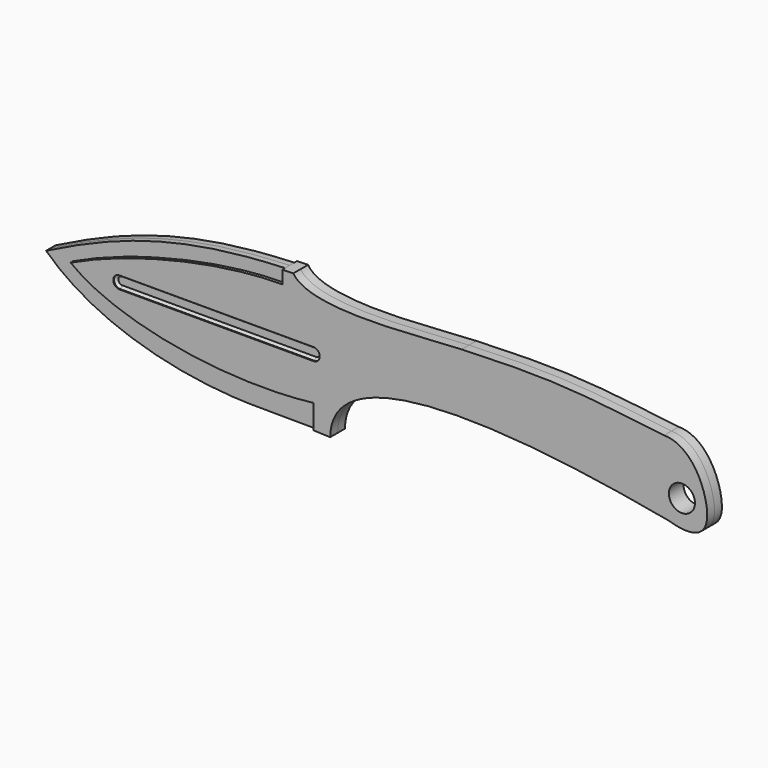
from build123d import *

# Parameters (mm, degrees)
F0_R     = 4.5078911523
F1_DEPTH = 3.175
F2_DEPTH = 2.032
F3_SIZE  = 0.8128
F4_DEPTH = 2.032


with BuildPart() as f1:
    # F0 (on Front) → F1 (new body, symmetric)
    with BuildSketch(Plane.XZ):
        with BuildLine():
            Line((-12.7, 37.1539426299), (-16.5483634919, 37.0321285824))
            Line((-16.5483634919, 37.0321285824), (-16.5483634919, 32.5395166874))
            add(Edge.make_bspline(
                [(-89.6837934852, 15.3515776619), (-70.5197155476, 24.6142111719), (-40.1840545237, 32.5395166874), (-16.5483634919, 32.5395166874)],
                knots=[0, 0, 0, 0, 75.1279998951, 75.1279998951, 75.1279998951, 75.1279998951], degree=3))
            add(Edge.make_bspline(
                [(-89.6837934852, 15.3515776619), (-73.0749294162, 2.4758265486), (-35.1310288534, -3.4930929542), (-5.7461196557, 0)],
                knots=[0, 0, 0, 0, 85.3299714322, 85.3299714322, 85.3299714322, 85.3299714322], degree=3))
            Line((-5.7461196557, 0), (-5.7461196557, -8.3546908572))
            add(Edge.make_bspline(
                [(-5.7461196557, -8.3546908572), (-3.9324804497, -8.403058144), (-2.0242283828, -8.4711340621), (0, -8.5660573701)],
                knots=[0.9484881406, 0.9484881406, 0.9484881406, 0.9484881406, 1, 1, 1, 1], degree=3))
            add(Edge.make_bspline(
                [(0, -8.5660573701), (0.2505557549, 0), (4.9891874099, 25.1308427086), (116.84, 4.123268791)],
                knots=[0, 0, 0, 0, 117.5270377336, 117.5270377336, 117.5270377336, 117.5270377336], degree=3))
            add(Edge.make_bspline(
                [(115.3515521604, 29.523268791), (122.3626523611, 29.4956252991), (132.2580267295, 16.9896472913), (130.5714420129, 0), (116.84, 4.123268791)],
                knots=[0, 0, 0, 0, 0.5223216622, 1, 1, 1, 1], degree=3))
            add(Edge.make_bspline(
                [(45.439671725, 32.9246893525), (77.6824429631, 34.1962501407), (85.773983987, 33.0161216226), (115.3515521604, 29.523268791)],
                knots=[0, 0, 0, 0, 69.9945761316, 69.9945761316, 69.9945761316, 69.9945761316], degree=3))
            add(Edge.make_bspline(
                [(-12.7, 37.1539426299), (-6.8683245444, 27.488068858), (34.4762634486, 32.667491585), (45.439671725, 32.9246893525)],
                knots=[0, 0, 0, 0, 58.293293024, 58.293293024, 58.293293024, 58.293293024], degree=3))
        make_face()
        with Locations((121.5164735913, 12.3797915876)):
            Circle(F0_R, mode=Mode.SUBTRACT)
        with BuildLine():
            ThreePointArc((-72.787091136, 12.7), (-74.9297025613, 14.8426114254), (-72.787091136, 16.9852228507))
            Line((-72.787091136, 16.9852228507), (-5.7461196557, 16.9852228507))
            ThreePointArc((-5.7461196557, 16.9852228507), (-3.6035082303, 14.8426114254), (-5.7461196557, 12.7))
            Line((-5.7461196557, 12.7), (-72.787091136, 12.7))
        make_face(mode=Mode.SUBTRACT)
    extrude(amount=F1_DEPTH, both=True)

    # F0 (on Front) → F2 (join, symmetric)
    with BuildSketch(Plane.XZ):
        with BuildLine():
            Line((-5.7461196557, 16.9852228507), (-72.787091136, 16.9852228507))
            ThreePointArc((-72.787091136, 16.9852228507), (-74.9297025613, 14.8426114254), (-72.787091136, 12.7))
            Line((-72.787091136, 12.7), (-5.7461196557, 12.7))
            ThreePointArc((-5.7461196557, 12.7), (-3.6035082303, 14.8426114254), (-5.7461196557, 16.9852228507))
        make_face()
    extrude(amount=F2_DEPTH, both=True)

    # F3
    f3_edges = [f1.edges().sort_by_distance(p)[0] for p in [
        (-39.266605, 2.032, 16.985223),
        (-74.929703, 2.032, 14.842611),
        (-39.266605, 2.032, 12.7),
        (-3.603508, 2.032, 14.842611),
        (-39.266605, -2.032, 16.985223),
        (-74.929703, -2.032, 14.842611),
        (-39.266605, -2.032, 12.7),
        (-3.603508, -2.032, 14.842611),
    ]]
    chamfer(f3_edges, length=F3_SIZE)


with BuildPart() as f4:
    # F0 (on Front) → F4 (new body, symmetric)
    with BuildSketch(Plane.XZ):
        with BuildLine():
            Line((-89.6837934852, 15.3515776619), (-99.06, 15.4687920451))
            add(Edge.make_bspline(
                [(-99.06, 15.4687920451), (-82.8389597692, 0), (-39.6847026689, -9.8562336065), (-19.5396852167, -7.9868352559), (-5.7461196557, -8.3546908572)],
                knots=[0, 0, 0, 0, 0.5567166084, 0.9484881406, 0.9484881406, 0.9484881406, 0.9484881406], degree=3))
            Line((-5.7461196557, -8.3546908572), (-5.7461196557, 0))
            add(Edge.make_bspline(
                [(-89.6837934852, 15.3515776619), (-73.0749294162, 2.4758265486), (-35.1310288534, -3.4930929542), (-5.7461196557, 0)],
                knots=[0, 0, 0, 0, 85.3299714322, 85.3299714322, 85.3299714322, 85.3299714322], degree=3))
        make_face()
        with BuildLine():
            add(Edge.make_bspline(
                [(-99.06, 15.4687920451), (-74.216040337, 28.1011594833), (-52.1198845092, 35.6695184857), (-16.5483634919, 37.0321285824)],
                knots=[0, 0, 0, 0, 88.4644885146, 88.4644885146, 88.4644885146, 88.4644885146], degree=3))
            Line((-99.06, 15.4687920451), (-89.6837934852, 15.3515776619))
            add(Edge.make_bspline(
                [(-89.6837934852, 15.3515776619), (-70.5197155476, 24.6142111719), (-40.1840545237, 32.5395166874), (-16.5483634919, 32.5395166874)],
                knots=[0, 0, 0, 0, 75.1279998951, 75.1279998951, 75.1279998951, 75.1279998951], degree=3))
            Line((-16.5483634919, 32.5395166874), (-16.5483634919, 37.0321285824))
        make_face()
    extrude(amount=F4_DEPTH, both=True)


solid = Compound([f1.part, f4.part])
